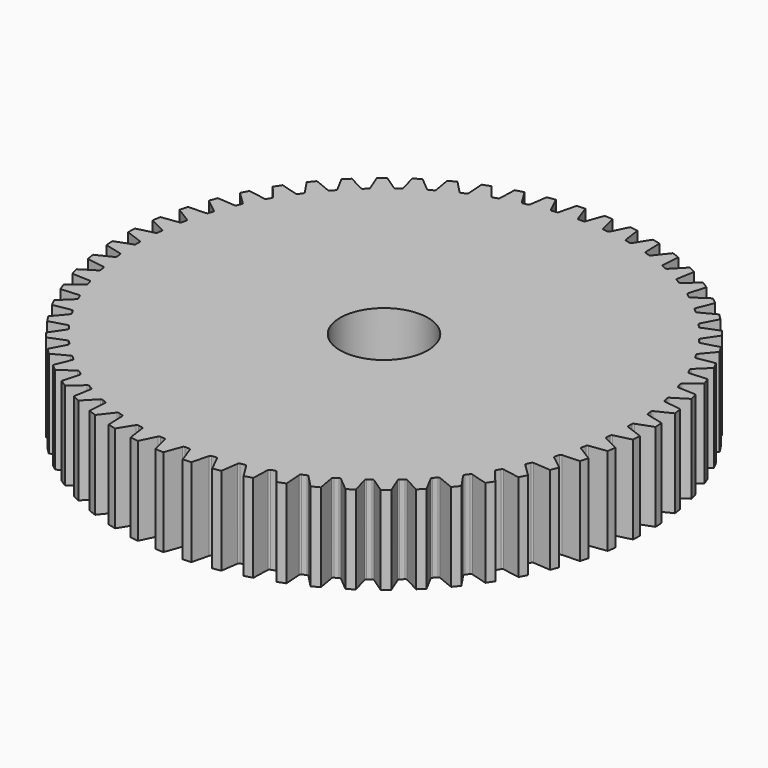
from build123d import *

# Parameters (mm, degrees)
F0_R            = 38.1
F1_DEPTH        = 12.7
F3_DEPTH        = 25.4
F3_COPIES_COUNT = 60
F4_R            = 0.254
F7_D            = 12.7
F7_DEPTH        = 25.4
F7_TIP          = 3.8154649308


# Not quite as in the source:
# - a feature of the source that left no trace in its solid (it failed there, or was rolled back) is left out
# - a pattern or mirror of a feature is missing from the dataset's text; its kind, count and spacing are read off the source's solid


with BuildPart() as f1:
    # F0 (on Top) → F1 (new body)
    with BuildSketch(Plane.XY):
        Circle(F0_R)
    extrude(amount=F1_DEPTH)

    # F2 (on face) → F3 (cut)
    with BuildSketch(Plane.XY.offset(12.7)):
        with BuildLine():
            Line((0.4784628608, 35.5442661897), (1.3993178947, 38.0742946019))
            ThreePointArc((1.3993178947, 38.0742946019), (0, 38.1), (-1.3993178947, 38.0742946019))
            Line((-1.3993178947, 38.0742946019), (-0.4784628608, 35.5442661897))
            Line((-0.4784628608, 35.5442661897), (0.4784628608, 35.5442661897))
        make_face()
    f3 = extrude(amount=-F3_DEPTH, mode=Mode.SUBTRACT)

    # F3_copies: F3 ×60 about axis
    f3_copies_axis = Axis((0, 0, 0), (0, 0, 1))
    for i in range(1, F3_COPIES_COUNT):
        add(f3.rotate(f3_copies_axis, i * 360 / F3_COPIES_COUNT), mode=Mode.SUBTRACT)

    # F4
    f4_edges = [f1.edges().sort_by_distance(p)[0] for p in [
        (-0.478463, 35.544266, 6.35),
        (0.478463, 35.544266, 6.35),
        (-6.922061, 34.867017, 6.35),
        (-4.191229, 35.299538, 6.35),
        (3.239546, 35.399564, 6.35),
        (4.191229, 35.299538, 6.35),
        (6.922061, 34.867017, 6.35),
        (7.858076, 34.668061, 6.35),
        (10.528737, 33.952459, 6.35),
        (11.438828, 33.656753, 6.35),
        (14.020058, 32.665911, 6.35),
        (14.894253, 32.276695, 6.35),
        (17.357772, 31.021469, 6.35),
        (18.186494, 30.543006, 6.35),
        (20.505311, 29.037149, 6.35),
        (21.27948, 28.474682, 6.35),
        (23.428189, 26.734692, 6.35),
        (24.139324, 26.094383, 6.35),
        (26.094383, 24.139324, 6.35),
        (26.734692, 23.428189, 6.35),
        (28.474682, 21.27948, 6.35),
        (29.037149, 20.505311, 6.35),
        (30.543006, 18.186494, 6.35),
        (31.021469, 17.357772, 6.35),
        (32.276695, 14.894253, 6.35),
        (32.665911, 14.020058, 6.35),
        (33.656753, 11.438828, 6.35),
        (33.952459, 10.528737, 6.35),
        (34.668061, 7.858076, 6.35),
        (34.867017, 6.922061, 6.35),
        (35.299538, 4.191229, 6.35),
        (35.399564, 3.239546, 6.35),
        (35.544266, 0.478463, 6.35),
        (35.544266, -0.478463, 6.35),
        (35.399564, -3.239546, 6.35),
        (35.299538, -4.191229, 6.35),
        (34.867017, -6.922061, 6.35),
        (34.668061, -7.858076, 6.35),
        (33.952459, -10.528737, 6.35),
        (33.656753, -11.438828, 6.35),
        (32.665911, -14.020058, 6.35),
        (32.276695, -14.894253, 6.35),
        (31.021469, -17.357772, 6.35),
        (30.543006, -18.186494, 6.35),
        (29.037149, -20.505311, 6.35),
        (28.474682, -21.27948, 6.35),
        (26.734692, -23.428189, 6.35),
        (26.094383, -24.139324, 6.35),
        (24.139324, -26.094383, 6.35),
        (23.428189, -26.734692, 6.35),
        (21.27948, -28.474682, 6.35),
        (20.505311, -29.037149, 6.35),
        (18.186494, -30.543006, 6.35),
        (17.357772, -31.021469, 6.35),
        (14.894253, -32.276695, 6.35),
        (14.020058, -32.665911, 6.35),
        (11.438828, -33.656753, 6.35),
        (10.528737, -33.952459, 6.35),
        (7.858076, -34.668061, 6.35),
        (6.922061, -34.867017, 6.35),
        (4.191229, -35.299538, 6.35),
        (3.239546, -35.399564, 6.35),
        (0.478463, -35.544266, 6.35),
        (-0.478463, -35.544266, 6.35),
        (-3.239546, -35.399564, 6.35),
        (-4.191229, -35.299538, 6.35),
        (-6.922061, -34.867017, 6.35),
        (-7.858076, -34.668061, 6.35),
        (-10.528737, -33.952459, 6.35),
        (-11.438828, -33.656753, 6.35),
        (-14.020058, -32.665911, 6.35),
        (-14.894253, -32.276695, 6.35),
        (-17.357772, -31.021469, 6.35),
        (-18.186494, -30.543006, 6.35),
        (-20.505311, -29.037149, 6.35),
        (-21.27948, -28.474682, 6.35),
        (-23.428189, -26.734692, 6.35),
        (-24.139324, -26.094383, 6.35),
        (-26.094383, -24.139324, 6.35),
        (-26.734692, -23.428189, 6.35),
        (-28.474682, -21.27948, 6.35),
        (-29.037149, -20.505311, 6.35),
        (-30.543006, -18.186494, 6.35),
        (-31.021469, -17.357772, 6.35),
        (-32.276695, -14.894253, 6.35),
        (-32.665911, -14.020058, 6.35),
        (-33.656753, -11.438828, 6.35),
        (-33.952459, -10.528737, 6.35),
        (-34.668061, -7.858076, 6.35),
        (-34.867017, -6.922061, 6.35),
        (-35.299538, -4.191229, 6.35),
        (-35.399564, -3.239546, 6.35),
        (-35.544266, -0.478463, 6.35),
        (-35.544266, 0.478463, 6.35),
        (-35.399564, 3.239546, 6.35),
        (-35.299538, 4.191229, 6.35),
        (-34.867017, 6.922061, 6.35),
        (-34.668061, 7.858076, 6.35),
        (-33.952459, 10.528737, 6.35),
        (-33.656753, 11.438828, 6.35),
        (-32.665911, 14.020058, 6.35),
        (-32.276695, 14.894253, 6.35),
        (-31.021469, 17.357772, 6.35),
        (-30.543006, 18.186494, 6.35),
        (-29.037149, 20.505311, 6.35),
        (-28.474682, 21.27948, 6.35),
        (-26.734692, 23.428189, 6.35),
        (-26.094383, 24.139324, 6.35),
        (-24.139324, 26.094383, 6.35),
        (-23.428189, 26.734692, 6.35),
        (-21.27948, 28.474682, 6.35),
        (-20.505311, 29.037149, 6.35),
        (-18.186494, 30.543006, 6.35),
        (-17.357772, 31.021469, 6.35),
        (-14.894253, 32.276695, 6.35),
        (-14.020058, 32.665911, 6.35),
        (-11.438828, 33.656753, 6.35),
        (-10.528737, 33.952459, 6.35),
        (-7.858076, 34.668061, 6.35),
        (-3.239546, 35.399564, 6.35),
    ]]
    fillet(f4_edges, radius=F4_R)

    # F7
    with Locations(Plane.XY.offset(12.7)):
        with Locations((0, 0)):
            Hole(F7_D / 2, depth=F7_DEPTH)
            with Locations((0, 0, -(F7_DEPTH + F7_TIP / 2))):  # 118° drill point
                Cone(0, F7_D / 2, F7_TIP, mode=Mode.SUBTRACT)


solid = f1.part
